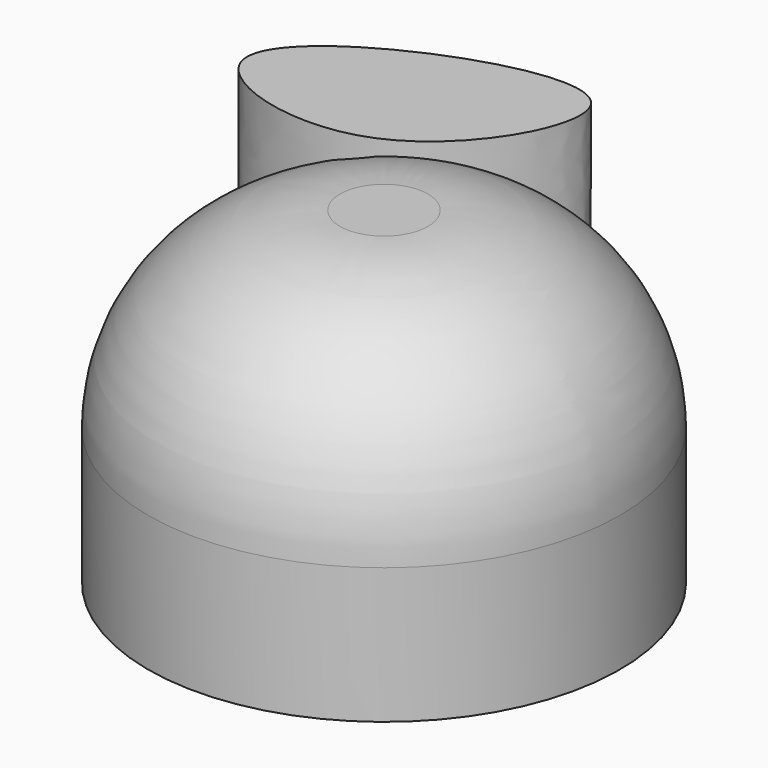
from build123d import *

# Parameters (mm, degrees)
F0_R     = 43.7038461673
F1_DEPTH = 60.706
F3_D     = 6.35
F6_DEPTH = 53.4


# Not quite as in the source:
# - a fillet or chamfer that OpenCascade refuses, or shapes differently, is made with other operations: its cross-section is extruded or revolved along the edge and cut away or added


with BuildPart() as f1:
    # F0 (on Top) → F1 (new body)
    with BuildSketch(Plane.XY):
        Circle(F0_R)
    extrude(amount=F1_DEPTH)

    # F3 (through all)
    with Locations(Plane.XY.offset(60.706)):
        with Locations((-18.8752301037, 16.5682565421)):
            Hole(F3_D / 2)

    # F4: fillet of radius 35.5661942009 on 1 edges, made by hand

    # F4_s1 → F4_t2 (revolve, cut)
    with BuildSketch(Plane.XZ):
        with BuildLine():
            ThreePointArc((43.7038461673, 25.1398057991), (33.2867490669, 50.2889028996), (8.1376519665, 60.706))
            Line((8.1376519665, 60.706), (43.7038461673, 60.706))
            Line((43.7038461673, 60.706), (43.7038461673, 25.1398057991))
        make_face()
    revolve(axis=Axis((0, 0, 60.706), (0, 0, 1)), mode=Mode.SUBTRACT)

    # F5 (on Top) → F6 (join)
    with BuildSketch(Plane.XY):
        with BuildLine():
            add(Edge.make_bspline(
                [(-53.932659328, 34.245159477), (-56.092631888, 40.1822694312), (-37.6274698884, 55.2882292442), (5.9776268015, 64.529029477), (-19.7151067113, 17.6140446523), (-51.5549907385, 27.7096691138), (-53.932659328, 34.245159477)],
                knots=[0, 0, 0, 0, 0.2312508113, 0.4835795296, 0.7454422336, 1, 1, 1, 1], degree=3))
        make_face()
    extrude(amount=F6_DEPTH)


solid = f1.part
